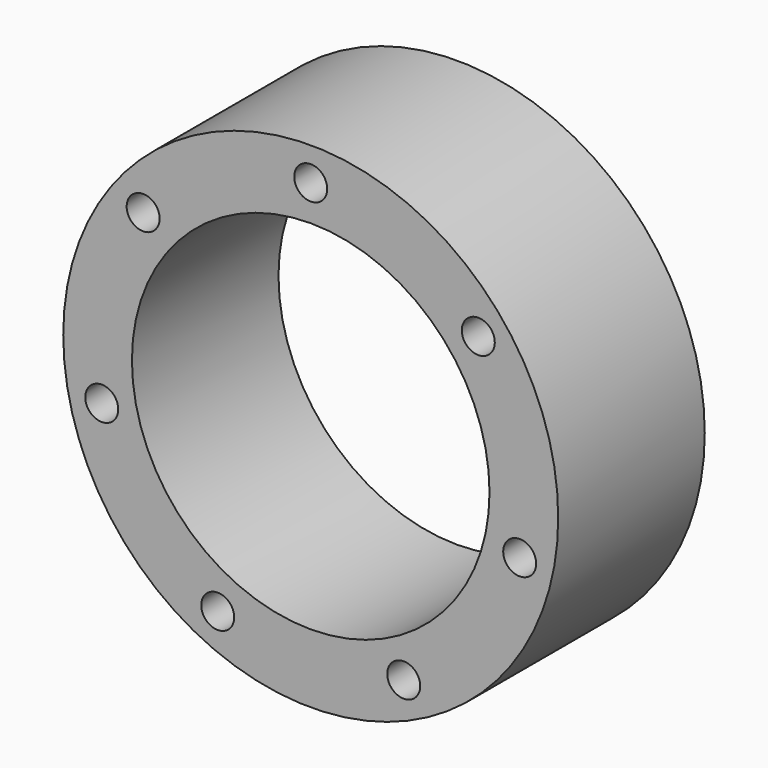
from build123d import *

# Parameters (mm, degrees)
F0_W            = 4.7625
F0_H            = 12.7
F3_R            = 1.143
F4_DEPTH        = 12.7
F4_COPIES_COUNT = 7


# Not quite as in the source:
# - a pattern or mirror of a feature is missing from the dataset's text; its kind, count and spacing are read off the source's solid


with BuildPart() as f1:
    # F0 (on Top) → F1 (revolve)
    with BuildSketch(Plane.XY):
        with Locations((14.77645, 0)):
            Rectangle(F0_W, F0_H)
    revolve(axis=Axis((0, -1.5469156838, 0), (0, -1, 0)))

    # F3 (on face) → F4 (cut, through all)
    with BuildSketch(Plane.XZ.offset(6.35)):
        with Locations((0, 14.859)):
            Circle(F3_R)
    f4 = extrude(amount=-F4_DEPTH, mode=Mode.SUBTRACT)

    # F4_copies: F4 ×7 about axis
    f4_copies_axis = Axis((0, 0, 0), (0, 1, 0))
    for i in range(1, F4_COPIES_COUNT):
        add(f4.rotate(f4_copies_axis, i * 360 / F4_COPIES_COUNT), mode=Mode.SUBTRACT)


solid = f1.part
